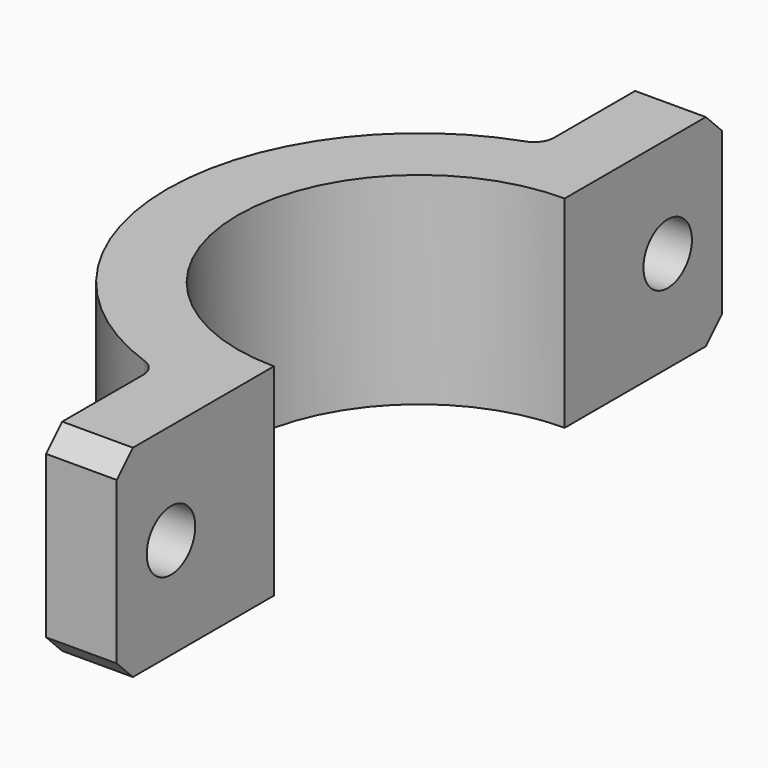
from build123d import *

# Parameters (mm, degrees)
F1_DEPTH = 20
F3_D     = 6
F4_SIZE  = 2
F5_R     = 2
F7_D     = 12
F7_DEPTH = 12
F7_TIP   = 3.6051637142
F9_D     = 12
F9_DEPTH = 12
F9_TIP   = 3.6051637142


# Not quite as in the source:
# - a feature names something its author has since deleted; it is built from what else it names


with BuildPart() as f1:
    # F0 (on Top) → F1 (new body)
    with BuildSketch(Plane.XY):
        with BuildLine():
            Line((0, 18), (0, 22.5))
            Line((0, 22.5), (0, 37.4649850279))
            Line((0, 37.4649850279), (-7, 37.4649850279))
            Line((-7, 37.4649850279), (-7, 24))
            ThreePointArc((-7, 24), (-25, 0), (-7, -24))
            Line((-7, -24), (-7, -37.4649850279))
            Line((-7, -37.4649850279), (0, -37.4649850279))
            Line((0, -37.4649850279), (0, -22.5))
            Line((0, -22.5), (0, -18))
            ThreePointArc((0, -18), (-18, 0), (0, 18))
        make_face()
    extrude(amount=F1_DEPTH)

    # F3 (through all)
    with Locations(Plane.YZ):
        with Locations((-30.75, 10), (30.75, 10)):
            Hole(F3_D / 2)

    # F4
    f4_edges = [f1.edges().sort_by_distance(p)[0] for p in [
        (-3.5, -37.464985, 20),
        (-3.5, -37.464985, 0),
        (-3.5, 37.464985, 20),
        (-3.5, 37.464985, 0),
    ]]
    chamfer(f4_edges, length=F4_SIZE)

    # F5
    f5_edges = [f1.edges().sort_by_distance(p)[0] for p in [
        (-7, -24, 10),
        (-7, 24, 10),
    ]]
    fillet(f5_edges, radius=F5_R)

    # F7 (one way)
    with BuildSketch(Plane(origin=(-7, 0, 0), x_dir=(0, -1, 0), z_dir=(1, 0, 0))):
        with Locations((30.75, -10)):
            Circle(F7_D / 2)
    extrude(amount=-F7_DEPTH, mode=Mode.SUBTRACT)
    with Locations(Plane(origin=(-7, 0, 0), x_dir=(0, -1, 0), z_dir=(1, 0, 0))):
        with Locations((30.75, -10)):
            with Locations((0, 0, -(F7_DEPTH + F7_TIP / 2))):  # 118° drill point
                Cone(0, F7_D / 2, F7_TIP, mode=Mode.SUBTRACT)

    # F9 (one way)
    with BuildSketch(Plane(origin=(-7, 0, 0), x_dir=(0, -1, 0), z_dir=(1, 0, 0))):
        with Locations((-30.75, -10)):
            Circle(F9_D / 2)
    extrude(amount=-F9_DEPTH, mode=Mode.SUBTRACT)
    with Locations(Plane(origin=(-7, 0, 0), x_dir=(0, -1, 0), z_dir=(1, 0, 0))):
        with Locations((-30.75, -10)):
            with Locations((0, 0, -(F9_DEPTH + F9_TIP / 2))):  # 118° drill point
                Cone(0, F9_D / 2, F9_TIP, mode=Mode.SUBTRACT)


solid = f1.part
